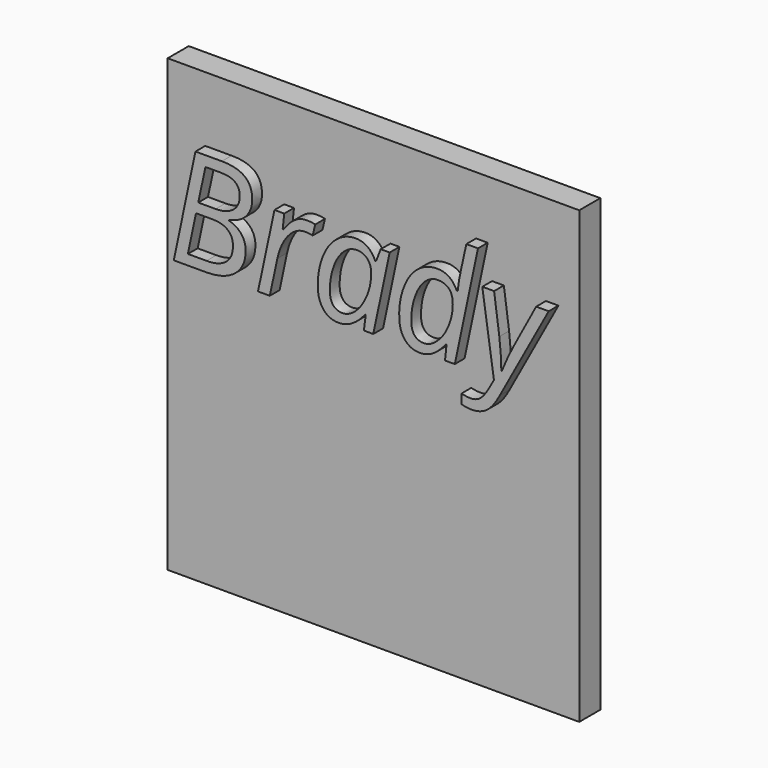
from build123d import *

# Parameters (mm, degrees)
F0_W         = 107.1351841092
F0_H         = 117.2422766685
F1_DEPTH     = 6.858
F2_TEXT_SIZE = 37.4929366315
F3_DEPTH     = 3.175


# Not quite as in the source:
# - a feature names something its author has since deleted; it is built from what else it names
# - Text() gives the source's letters only with a copy of the font that has no kerning and outlines rounded to 1/6400 em; it was checked with that copy


with BuildPart() as f1:
    # F0 (on Front) → F1 (new body)
    with BuildSketch(Plane.XZ):
        with Locations((7.5430907309, 10.119907558)):
            Rectangle(F0_W, F0_H)
    extrude(amount=F1_DEPTH)

    # F2 (on face) → F3 (join)
    with BuildSketch(Plane.XZ.offset(6.858)):
        with Locations((-43.4761595915, 25.0716925852)):
            Text('Brady', F2_TEXT_SIZE, font='Open Sans', font_style=FontStyle.ITALIC, text_align=(TextAlign.LEFT, TextAlign.BOTTOM))
    extrude(amount=F3_DEPTH)


solid = f1.part
